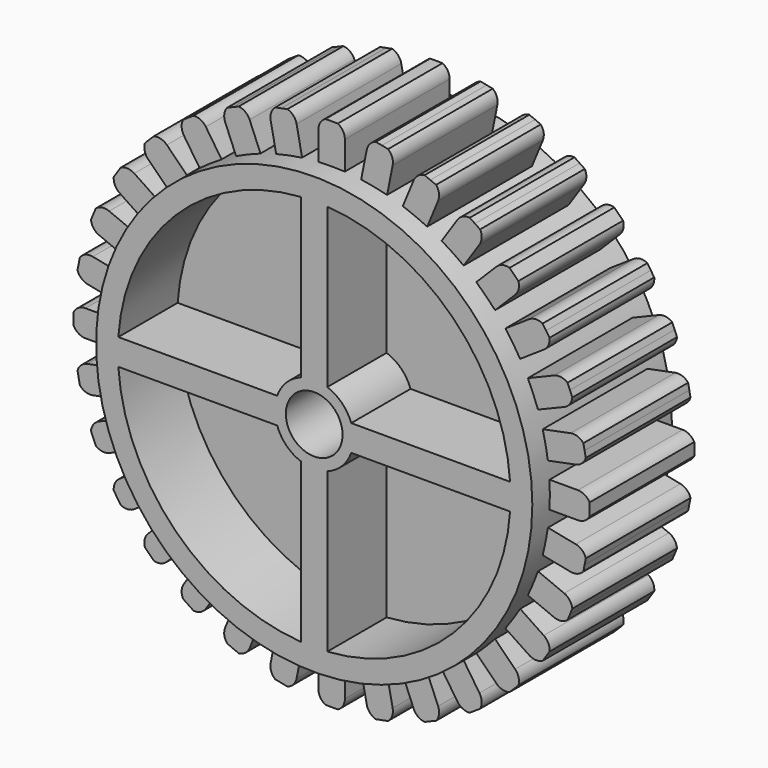
from build123d import *

# Parameters (mm, degrees)
F0_R      = 50
F1_DEPTH  = 20
F3_DEPTH  = 17
F5_DEPTH  = 17
F7_DEPTH  = 15
F8_R      = 9
F8_R_2    = 6.5
F9_DEPTH  = 20
F10_R     = 6.5
F11_DEPTH = 21


# Not quite as in the source:
# - a feature names something its author has since deleted; it is built from what else it names


with BuildPart() as f1:
    # F0 (on Front) → F1 (new body, symmetric)
    with BuildSketch(Plane.XZ):
        Circle(F0_R)
    extrude(amount=F1_DEPTH, both=True)

    # F2 (on face) → F3 (cut)
    with BuildSketch(Plane.XZ.offset(20)):
        with BuildLine():
            Line((-3, -3), (-44.8998886413, -3))
            ThreePointArc((-44.8998886413, -3), (-31.8198051534, -31.8198051534), (-3, -44.8998886413))
            Line((-3, -44.8998886413), (-3, -3))
        make_face()
        with BuildLine():
            ThreePointArc((-3, 44.8998886413), (-31.8198051534, 31.8198051534), (-44.8998886413, 3))
            Line((-44.8998886413, 3), (-3.2378670737, 3))
            Line((-3.2378670737, 3), (-3, 3.2378670737))
            Line((-3, 3.2378670737), (-3, 44.8998886413))
        make_face()
        Polygon((-3, 3.2378670737), (-3.2378670737, 3), (-3, 3), align=None)
        with BuildLine():
            ThreePointArc((44.8998886413, 3), (31.8198051534, 31.8198051534), (3, 44.8998886413))
            Line((3, 44.8998886413), (3, 3))
            Line((3, 3), (44.8998886413, 3))
        make_face()
        with BuildLine():
            Line((44.8998886413, -3), (3, -3))
            Line((3, -3), (3, -44.8998886413))
            ThreePointArc((3, -44.8998886413), (31.8198051534, -31.8198051534), (44.8998886413, -3))
        make_face()
    extrude(amount=-F3_DEPTH, mode=Mode.SUBTRACT)

    # F4 (on face) → F5 (cut)
    with BuildSketch(Plane(origin=(0, 20, 0), x_dir=(-1, 0, 0), z_dir=(0, 1, 0))):
        with BuildLine():
            Line((3, -3), (3, -44.8998886413))
            ThreePointArc((3, -44.8998886413), (31.8198051534, -31.8198051534), (44.8998886413, -3))
            Line((44.8998886413, -3), (3, -3))
        make_face()
        with BuildLine():
            Line((3, 3), (44.8998886413, 3))
            ThreePointArc((44.8998886413, 3), (31.8198051534, 31.8198051534), (3, 44.8998886413))
            Line((3, 44.8998886413), (3, 3))
        make_face()
        with BuildLine():
            ThreePointArc((-44.8998886413, -3), (-31.8198051534, -31.8198051534), (-3, -44.8998886413))
            Line((-3, -44.8998886413), (-3, -3))
            Line((-3, -3), (-44.8998886413, -3))
        make_face()
        with BuildLine():
            Line((-44.8998886413, 3), (-3, 3))
            Line((-3, 3), (-3, 44.8998886413))
            ThreePointArc((-3, 44.8998886413), (-31.8198051534, 31.8198051534), (-44.8998886413, 3))
        make_face()
    extrude(amount=-F5_DEPTH, mode=Mode.SUBTRACT)

    # F6 (on Front) → F7 (join, symmetric)
    with BuildSketch(Plane.XZ):
        with BuildLine():
            Line((-3.0323624939, 56.4412474632), (-3.0323624939, 49.947373569))
            Line((-3.0323624939, 49.947373569), (0, 49.947373569))
            Line((0, 49.947373569), (3.0323624939, 49.947373569))
            Line((3.0323624939, 49.947373569), (3.0323624939, 56.4412474632))
            ThreePointArc((3.0323624939, 56.4412474632), (2.5992583475, 58.0030023535), (1.4236640997, 59.1186347766))
            Line((1.4236640997, 59.1186347766), (0, 59.1186347766))
            Line((0, 59.1186347766), (-1.4236640997, 59.1186347766))
            ThreePointArc((-1.4236640997, 59.1186347766), (-2.5992583475, 58.0030023535), (-3.0323624939, 56.4412474632))
        make_face()
        with BuildLine():
            Line((-13.9852376415, 54.7651601441), (-12.7183456923, 48.3960642159))
            Line((-12.7183456923, 48.3960642159), (-9.7442491934, 48.9876487913))
            Line((-9.7442491934, 48.9876487913), (-6.7701526945, 49.5792333667))
            Line((-6.7701526945, 49.5792333667), (-8.0370446437, 55.9483292949))
            ThreePointArc((-8.0370446437, 55.9483292949), (-8.7665100798, 57.3955810756), (-10.1371647025, 58.2604298741))
            Line((-10.1371647025, 58.2604298741), (-11.5334734957, 57.9826867864))
            Line((-11.5334734957, 57.9826867864), (-12.9297822889, 57.7049436988))
            ThreePointArc((-12.9297822889, 57.7049436988), (-13.8651387343, 56.3814007795), (-13.9852376415, 54.7651601441))
        make_face()
        with BuildLine():
            Line((-24.4006679495, 50.9844784333), (-21.9155699983, 44.9849212558))
            Line((-21.9155699983, 44.9849212558), (-19.114032355, 46.1453561431))
            Line((-19.114032355, 46.1453561431), (-16.3124947117, 47.3057910305))
            Line((-16.3124947117, 47.3057910305), (-18.7975926629, 53.305348208))
            ThreePointArc((-18.7975926629, 53.305348208), (-19.7953864411, 54.5824798047), (-21.3084279502, 55.1633093243))
            Line((-21.3084279502, 55.1633093243), (-22.6237220731, 54.6184966601))
            Line((-22.6237220731, 54.6184966601), (-23.9390161959, 54.0736839959))
            ThreePointArc((-23.9390161959, 54.0736839959), (-24.5981896151, 52.5930935926), (-24.4006679495, 50.9844784333))
        make_face()
        with BuildLine():
            Line((-33.8783942723, 45.2444918088), (-30.2705912396, 39.8450329996))
            Line((-30.2705912396, 39.8450329996), (-27.7492739725, 41.529723337))
            Line((-27.7492739725, 41.529723337), (-25.2279567053, 43.2144136743))
            Line((-25.2279567053, 43.2144136743), (-28.8357597379, 48.6138724835))
            ThreePointArc((-28.8357597379, 48.6138724835), (-30.0635372029, 49.6718044451), (-31.6608202616, 49.9462937332))
            Line((-31.6608202616, 49.9462937332), (-32.8445536986, 49.1553483376))
            Line((-32.8445536986, 49.1553483376), (-34.0282871357, 48.364402942))
            ThreePointArc((-34.0282871357, 48.364402942), (-34.3859458639, 46.7836633135), (-33.8783942723, 45.2444918088))
        make_face()
        with BuildLine():
            Line((-42.0541929024, 37.7657847374), (-37.4623306356, 33.1739224706))
            Line((-37.4623306356, 33.1739224706), (-35.3181265531, 35.3181265531))
            Line((-35.3181265531, 35.3181265531), (-33.1739224706, 37.4623306356))
            Line((-33.1739224706, 37.4623306356), (-37.7657847374, 42.0541929024))
            ThreePointArc((-37.7657847374, 42.0541929024), (-39.1763630898, 42.852269497), (-40.796505006, 42.809870084))
            Line((-40.796505006, 42.809870084), (-41.803187545, 41.803187545))
            Line((-41.803187545, 41.803187545), (-42.809870084, 40.796505006))
            ThreePointArc((-42.809870084, 40.796505006), (-42.852269497, 39.1763630898), (-42.0541929024, 37.7657847374))
        make_face()
        with BuildLine():
            Line((-48.6138724835, 28.8357597379), (-43.2144136743, 25.2279567053))
            Line((-43.2144136743, 25.2279567053), (-41.529723337, 27.7492739725))
            Line((-41.529723337, 27.7492739725), (-39.8450329996, 30.2705912396))
            Line((-39.8450329996, 30.2705912396), (-45.2444918088, 33.8783942723))
            ThreePointArc((-45.2444918088, 33.8783942723), (-46.7836633135, 34.3859458639), (-48.364402942, 34.0282871357))
            Line((-48.364402942, 34.0282871357), (-49.1553483376, 32.8445536986))
            Line((-49.1553483376, 32.8445536986), (-49.9462937332, 31.6608202616))
            ThreePointArc((-49.9462937332, 31.6608202616), (-49.6718044451, 30.0635372029), (-48.6138724835, 28.8357597379))
        make_face()
        with BuildLine():
            Line((-53.305348208, 18.7975926629), (-47.3057910305, 16.3124947117))
            Line((-47.3057910305, 16.3124947117), (-46.1453561431, 19.114032355))
            Line((-46.1453561431, 19.114032355), (-44.9849212558, 21.9155699983))
            Line((-44.9849212558, 21.9155699983), (-50.9844784333, 24.4006679495))
            ThreePointArc((-50.9844784333, 24.4006679495), (-52.5930935926, 24.5981896151), (-54.0736839959, 23.9390161959))
            Line((-54.0736839959, 23.9390161959), (-54.6184966601, 22.6237220731))
            Line((-54.6184966601, 22.6237220731), (-55.1633093243, 21.3084279502))
            ThreePointArc((-55.1633093243, 21.3084279502), (-54.5824798047, 19.7953864411), (-53.305348208, 18.7975926629))
        make_face()
        with BuildLine():
            Line((-55.9483292949, 8.0370446437), (-49.5792333667, 6.7701526945))
            Line((-49.5792333667, 6.7701526945), (-48.9876487913, 9.7442491934))
            Line((-48.9876487913, 9.7442491934), (-48.3960642159, 12.7183456923))
            Line((-48.3960642159, 12.7183456923), (-54.7651601441, 13.9852376415))
            ThreePointArc((-54.7651601441, 13.9852376415), (-56.3814007795, 13.8651387343), (-57.7049436988, 12.9297822889))
            Line((-57.7049436988, 12.9297822889), (-57.9826867864, 11.5334734957))
            Line((-57.9826867864, 11.5334734957), (-58.2604298741, 10.1371647025))
            ThreePointArc((-58.2604298741, 10.1371647025), (-57.3955810756, 8.7665100798), (-55.9483292949, 8.0370446437))
        make_face()
        with BuildLine():
            Line((-56.4412474632, -3.0323624939), (-49.947373569, -3.0323624939))
            Line((-49.947373569, -3.0323624939), (-49.947373569, 0))
            Line((-49.947373569, 0), (-49.947373569, 3.0323624939))
            Line((-49.947373569, 3.0323624939), (-56.4412474632, 3.0323624939))
            ThreePointArc((-56.4412474632, 3.0323624939), (-58.0030023535, 2.5992583475), (-59.1186347766, 1.4236640997))
            Line((-59.1186347766, 1.4236640997), (-59.1186347766, 0))
            Line((-59.1186347766, 0), (-59.1186347766, -1.4236640997))
            ThreePointArc((-59.1186347766, -1.4236640997), (-58.0030023535, -2.5992583475), (-56.4412474632, -3.0323624939))
        make_face()
        with BuildLine():
            Line((-54.7651601441, -13.9852376415), (-48.3960642159, -12.7183456923))
            Line((-48.3960642159, -12.7183456923), (-48.9876487913, -9.7442491934))
            Line((-48.9876487913, -9.7442491934), (-49.5792333667, -6.7701526945))
            Line((-49.5792333667, -6.7701526945), (-55.9483292949, -8.0370446437))
            ThreePointArc((-55.9483292949, -8.0370446437), (-57.3955810756, -8.7665100798), (-58.2604298741, -10.1371647025))
            Line((-58.2604298741, -10.1371647025), (-57.9826867864, -11.5334734957))
            Line((-57.9826867864, -11.5334734957), (-57.7049436988, -12.9297822889))
            ThreePointArc((-57.7049436988, -12.9297822889), (-56.3814007795, -13.8651387343), (-54.7651601441, -13.9852376415))
        make_face()
        with BuildLine():
            Line((-50.9844784333, -24.4006679495), (-44.9849212558, -21.9155699983))
            Line((-44.9849212558, -21.9155699983), (-46.1453561431, -19.114032355))
            Line((-46.1453561431, -19.114032355), (-47.3057910305, -16.3124947117))
            Line((-47.3057910305, -16.3124947117), (-53.305348208, -18.7975926629))
            ThreePointArc((-53.305348208, -18.7975926629), (-54.5824798047, -19.7953864411), (-55.1633093243, -21.3084279502))
            Line((-55.1633093243, -21.3084279502), (-54.6184966601, -22.6237220731))
            Line((-54.6184966601, -22.6237220731), (-54.0736839959, -23.9390161959))
            ThreePointArc((-54.0736839959, -23.9390161959), (-52.5930935926, -24.5981896151), (-50.9844784333, -24.4006679495))
        make_face()
        with BuildLine():
            Line((-45.2444918088, -33.8783942723), (-39.8450329996, -30.2705912396))
            Line((-39.8450329996, -30.2705912396), (-41.529723337, -27.7492739725))
            Line((-41.529723337, -27.7492739725), (-43.2144136743, -25.2279567053))
            Line((-43.2144136743, -25.2279567053), (-48.6138724835, -28.8357597379))
            ThreePointArc((-48.6138724835, -28.8357597379), (-49.6718044451, -30.0635372029), (-49.9462937332, -31.6608202616))
            Line((-49.9462937332, -31.6608202616), (-49.1553483376, -32.8445536986))
            Line((-49.1553483376, -32.8445536986), (-48.364402942, -34.0282871357))
            ThreePointArc((-48.364402942, -34.0282871357), (-46.7836633135, -34.3859458639), (-45.2444918088, -33.8783942723))
        make_face()
        with BuildLine():
            Line((-37.7657847374, -42.0541929024), (-33.1739224706, -37.4623306356))
            Line((-33.1739224706, -37.4623306356), (-35.3181265531, -35.3181265531))
            Line((-35.3181265531, -35.3181265531), (-37.4623306356, -33.1739224706))
            Line((-37.4623306356, -33.1739224706), (-42.0541929024, -37.7657847374))
            ThreePointArc((-42.0541929024, -37.7657847374), (-42.852269497, -39.1763630898), (-42.809870084, -40.796505006))
            Line((-42.809870084, -40.796505006), (-41.803187545, -41.803187545))
            Line((-41.803187545, -41.803187545), (-40.796505006, -42.809870084))
            ThreePointArc((-40.796505006, -42.809870084), (-39.1763630898, -42.852269497), (-37.7657847374, -42.0541929024))
        make_face()
        with BuildLine():
            Line((-28.8357597379, -48.6138724835), (-25.2279567053, -43.2144136743))
            Line((-25.2279567053, -43.2144136743), (-27.7492739725, -41.529723337))
            Line((-27.7492739725, -41.529723337), (-30.2705912396, -39.8450329996))
            Line((-30.2705912396, -39.8450329996), (-33.8783942723, -45.2444918088))
            ThreePointArc((-33.8783942723, -45.2444918088), (-34.3859458639, -46.7836633135), (-34.0282871357, -48.364402942))
            Line((-34.0282871357, -48.364402942), (-32.8445536986, -49.1553483376))
            Line((-32.8445536986, -49.1553483376), (-31.6608202616, -49.9462937332))
            ThreePointArc((-31.6608202616, -49.9462937332), (-30.0635372029, -49.6718044451), (-28.8357597379, -48.6138724835))
        make_face()
        with BuildLine():
            Line((-18.7975926629, -53.305348208), (-16.3124947117, -47.3057910305))
            Line((-16.3124947117, -47.3057910305), (-19.114032355, -46.1453561431))
            Line((-19.114032355, -46.1453561431), (-21.9155699983, -44.9849212558))
            Line((-21.9155699983, -44.9849212558), (-24.4006679495, -50.9844784333))
            ThreePointArc((-24.4006679495, -50.9844784333), (-24.5981896151, -52.5930935926), (-23.9390161959, -54.0736839959))
            Line((-23.9390161959, -54.0736839959), (-22.6237220731, -54.6184966601))
            Line((-22.6237220731, -54.6184966601), (-21.3084279502, -55.1633093243))
            ThreePointArc((-21.3084279502, -55.1633093243), (-19.7953864411, -54.5824798047), (-18.7975926629, -53.305348208))
        make_face()
        with BuildLine():
            Line((-8.0370446437, -55.9483292949), (-6.7701526945, -49.5792333667))
            Line((-6.7701526945, -49.5792333667), (-9.7442491934, -48.9876487913))
            Line((-9.7442491934, -48.9876487913), (-12.7183456923, -48.3960642159))
            Line((-12.7183456923, -48.3960642159), (-13.9852376415, -54.7651601441))
            ThreePointArc((-13.9852376415, -54.7651601441), (-13.8651387343, -56.3814007795), (-12.9297822889, -57.7049436988))
            Line((-12.9297822889, -57.7049436988), (-11.5334734957, -57.9826867864))
            Line((-11.5334734957, -57.9826867864), (-10.1371647025, -58.2604298741))
            ThreePointArc((-10.1371647025, -58.2604298741), (-8.7665100798, -57.3955810756), (-8.0370446437, -55.9483292949))
        make_face()
        with BuildLine():
            Line((3.0323624939, -56.4412474632), (3.0323624939, -49.947373569))
            Line((3.0323624939, -49.947373569), (0, -49.947373569))
            Line((0, -49.947373569), (-3.0323624939, -49.947373569))
            Line((-3.0323624939, -49.947373569), (-3.0323624939, -56.4412474632))
            ThreePointArc((-3.0323624939, -56.4412474632), (-2.5992583475, -58.0030023535), (-1.4236640997, -59.1186347766))
            Line((-1.4236640997, -59.1186347766), (0, -59.1186347766))
            Line((0, -59.1186347766), (1.4236640997, -59.1186347766))
            ThreePointArc((1.4236640997, -59.1186347766), (2.5992583475, -58.0030023535), (3.0323624939, -56.4412474632))
        make_face()
        with BuildLine():
            Line((13.9852376415, -54.7651601441), (12.7183456923, -48.3960642159))
            Line((12.7183456923, -48.3960642159), (9.7442491934, -48.9876487913))
            Line((9.7442491934, -48.9876487913), (6.7701526945, -49.5792333667))
            Line((6.7701526945, -49.5792333667), (8.0370446437, -55.9483292949))
            ThreePointArc((8.0370446437, -55.9483292949), (8.7665100798, -57.3955810756), (10.1371647025, -58.2604298741))
            Line((10.1371647025, -58.2604298741), (11.5334734957, -57.9826867864))
            Line((11.5334734957, -57.9826867864), (12.9297822889, -57.7049436988))
            ThreePointArc((12.9297822889, -57.7049436988), (13.8651387343, -56.3814007795), (13.9852376415, -54.7651601441))
        make_face()
        with BuildLine():
            Line((24.4006679495, -50.9844784333), (21.9155699983, -44.9849212558))
            Line((21.9155699983, -44.9849212558), (19.114032355, -46.1453561431))
            Line((19.114032355, -46.1453561431), (16.3124947117, -47.3057910305))
            Line((16.3124947117, -47.3057910305), (18.7975926629, -53.305348208))
            ThreePointArc((18.7975926629, -53.305348208), (19.7953864411, -54.5824798047), (21.3084279502, -55.1633093243))
            Line((21.3084279502, -55.1633093243), (22.6237220731, -54.6184966601))
            Line((22.6237220731, -54.6184966601), (23.9390161959, -54.0736839959))
            ThreePointArc((23.9390161959, -54.0736839959), (24.5981896151, -52.5930935926), (24.4006679495, -50.9844784333))
        make_face()
        with BuildLine():
            Line((33.8783942723, -45.2444918088), (30.2705912396, -39.8450329996))
            Line((30.2705912396, -39.8450329996), (27.7492739725, -41.529723337))
            Line((27.7492739725, -41.529723337), (25.2279567053, -43.2144136743))
            Line((25.2279567053, -43.2144136743), (28.8357597379, -48.6138724835))
            ThreePointArc((28.8357597379, -48.6138724835), (30.0635372029, -49.6718044451), (31.6608202616, -49.9462937332))
            Line((31.6608202616, -49.9462937332), (32.8445536986, -49.1553483376))
            Line((32.8445536986, -49.1553483376), (34.0282871357, -48.364402942))
            ThreePointArc((34.0282871357, -48.364402942), (34.3859458639, -46.7836633135), (33.8783942723, -45.2444918088))
        make_face()
        with BuildLine():
            Line((42.0541929024, -37.7657847374), (37.4623306356, -33.1739224706))
            Line((37.4623306356, -33.1739224706), (35.3181265531, -35.3181265531))
            Line((35.3181265531, -35.3181265531), (33.1739224706, -37.4623306356))
            Line((33.1739224706, -37.4623306356), (37.7657847374, -42.0541929024))
            ThreePointArc((37.7657847374, -42.0541929024), (39.1763630898, -42.852269497), (40.796505006, -42.809870084))
            Line((40.796505006, -42.809870084), (41.803187545, -41.803187545))
            Line((41.803187545, -41.803187545), (42.809870084, -40.796505006))
            ThreePointArc((42.809870084, -40.796505006), (42.852269497, -39.1763630898), (42.0541929024, -37.7657847374))
        make_face()
        with BuildLine():
            Line((48.6138724835, -28.8357597379), (43.2144136743, -25.2279567053))
            Line((43.2144136743, -25.2279567053), (41.529723337, -27.7492739725))
            Line((41.529723337, -27.7492739725), (39.8450329996, -30.2705912396))
            Line((39.8450329996, -30.2705912396), (45.2444918088, -33.8783942723))
            ThreePointArc((45.2444918088, -33.8783942723), (46.7836633135, -34.3859458639), (48.364402942, -34.0282871357))
            Line((48.364402942, -34.0282871357), (49.1553483376, -32.8445536986))
            Line((49.1553483376, -32.8445536986), (49.9462937332, -31.6608202616))
            ThreePointArc((49.9462937332, -31.6608202616), (49.6718044451, -30.0635372029), (48.6138724835, -28.8357597379))
        make_face()
        with BuildLine():
            Line((53.305348208, -18.7975926629), (47.3057910305, -16.3124947117))
            Line((47.3057910305, -16.3124947117), (46.1453561431, -19.114032355))
            Line((46.1453561431, -19.114032355), (44.9849212558, -21.9155699983))
            Line((44.9849212558, -21.9155699983), (50.9844784333, -24.4006679495))
            ThreePointArc((50.9844784333, -24.4006679495), (52.5930935926, -24.5981896151), (54.0736839959, -23.9390161959))
            Line((54.0736839959, -23.9390161959), (54.6184966601, -22.6237220731))
            Line((54.6184966601, -22.6237220731), (55.1633093243, -21.3084279502))
            ThreePointArc((55.1633093243, -21.3084279502), (54.5824798047, -19.7953864411), (53.305348208, -18.7975926629))
        make_face()
        with BuildLine():
            Line((55.9483292949, -8.0370446437), (49.5792333667, -6.7701526945))
            Line((49.5792333667, -6.7701526945), (48.9876487913, -9.7442491934))
            Line((48.9876487913, -9.7442491934), (48.3960642159, -12.7183456923))
            Line((48.3960642159, -12.7183456923), (54.7651601441, -13.9852376415))
            ThreePointArc((54.7651601441, -13.9852376415), (56.3814007795, -13.8651387343), (57.7049436988, -12.9297822889))
            Line((57.7049436988, -12.9297822889), (57.9826867864, -11.5334734957))
            Line((57.9826867864, -11.5334734957), (58.2604298741, -10.1371647025))
            ThreePointArc((58.2604298741, -10.1371647025), (57.3955810756, -8.7665100798), (55.9483292949, -8.0370446437))
        make_face()
        with BuildLine():
            Line((56.4412474632, 3.0323624939), (49.947373569, 3.0323624939))
            Line((49.947373569, 3.0323624939), (49.947373569, 0))
            Line((49.947373569, 0), (49.947373569, -3.0323624939))
            Line((49.947373569, -3.0323624939), (56.4412474632, -3.0323624939))
            ThreePointArc((56.4412474632, -3.0323624939), (58.0030023535, -2.5992583475), (59.1186347766, -1.4236640997))
            Line((59.1186347766, -1.4236640997), (59.1186347766, 0))
            Line((59.1186347766, 0), (59.1186347766, 1.4236640997))
            ThreePointArc((59.1186347766, 1.4236640997), (58.0030023535, 2.5992583475), (56.4412474632, 3.0323624939))
        make_face()
        with BuildLine():
            Line((54.7651601441, 13.9852376415), (48.3960642159, 12.7183456923))
            Line((48.3960642159, 12.7183456923), (48.9876487913, 9.7442491934))
            Line((48.9876487913, 9.7442491934), (49.5792333667, 6.7701526945))
            Line((49.5792333667, 6.7701526945), (55.9483292949, 8.0370446437))
            ThreePointArc((55.9483292949, 8.0370446437), (57.3955810756, 8.7665100798), (58.2604298741, 10.1371647025))
            Line((58.2604298741, 10.1371647025), (57.9826867864, 11.5334734957))
            Line((57.9826867864, 11.5334734957), (57.7049436988, 12.9297822889))
            ThreePointArc((57.7049436988, 12.9297822889), (56.3814007795, 13.8651387343), (54.7651601441, 13.9852376415))
        make_face()
        with BuildLine():
            Line((50.9844784333, 24.4006679495), (44.9849212558, 21.9155699983))
            Line((44.9849212558, 21.9155699983), (46.1453561431, 19.114032355))
            Line((46.1453561431, 19.114032355), (47.3057910305, 16.3124947117))
            Line((47.3057910305, 16.3124947117), (53.305348208, 18.7975926629))
            ThreePointArc((53.305348208, 18.7975926629), (54.5824798047, 19.7953864411), (55.1633093243, 21.3084279502))
            Line((55.1633093243, 21.3084279502), (54.6184966601, 22.6237220731))
            Line((54.6184966601, 22.6237220731), (54.0736839959, 23.9390161959))
            ThreePointArc((54.0736839959, 23.9390161959), (52.5930935926, 24.5981896151), (50.9844784333, 24.4006679495))
        make_face()
        with BuildLine():
            Line((45.2444918088, 33.8783942723), (39.8450329996, 30.2705912396))
            Line((39.8450329996, 30.2705912396), (41.529723337, 27.7492739725))
            Line((41.529723337, 27.7492739725), (43.2144136743, 25.2279567053))
            Line((43.2144136743, 25.2279567053), (48.6138724835, 28.8357597379))
            ThreePointArc((48.6138724835, 28.8357597379), (49.6718044451, 30.0635372029), (49.9462937332, 31.6608202616))
            Line((49.9462937332, 31.6608202616), (49.1553483376, 32.8445536986))
            Line((49.1553483376, 32.8445536986), (48.364402942, 34.0282871357))
            ThreePointArc((48.364402942, 34.0282871357), (46.7836633135, 34.3859458639), (45.2444918088, 33.8783942723))
        make_face()
        with BuildLine():
            Line((37.7657847374, 42.0541929024), (33.1739224706, 37.4623306356))
            Line((33.1739224706, 37.4623306356), (35.3181265531, 35.3181265531))
            Line((35.3181265531, 35.3181265531), (37.4623306356, 33.1739224706))
            Line((37.4623306356, 33.1739224706), (42.0541929024, 37.7657847374))
            ThreePointArc((42.0541929024, 37.7657847374), (42.852269497, 39.1763630898), (42.809870084, 40.796505006))
            Line((42.809870084, 40.796505006), (41.803187545, 41.803187545))
            Line((41.803187545, 41.803187545), (40.796505006, 42.809870084))
            ThreePointArc((40.796505006, 42.809870084), (39.1763630898, 42.852269497), (37.7657847374, 42.0541929024))
        make_face()
        with BuildLine():
            Line((28.8357597379, 48.6138724835), (25.2279567053, 43.2144136743))
            Line((25.2279567053, 43.2144136743), (27.7492739725, 41.529723337))
            Line((27.7492739725, 41.529723337), (30.2705912396, 39.8450329996))
            Line((30.2705912396, 39.8450329996), (33.8783942723, 45.2444918088))
            ThreePointArc((33.8783942723, 45.2444918088), (34.3859458639, 46.7836633135), (34.0282871357, 48.364402942))
            Line((34.0282871357, 48.364402942), (32.8445536986, 49.1553483376))
            Line((32.8445536986, 49.1553483376), (31.6608202616, 49.9462937332))
            ThreePointArc((31.6608202616, 49.9462937332), (30.0635372029, 49.6718044451), (28.8357597379, 48.6138724835))
        make_face()
        with BuildLine():
            Line((18.7975926629, 53.305348208), (16.3124947117, 47.3057910305))
            Line((16.3124947117, 47.3057910305), (19.114032355, 46.1453561431))
            Line((19.114032355, 46.1453561431), (21.9155699983, 44.9849212558))
            Line((21.9155699983, 44.9849212558), (24.4006679495, 50.9844784333))
            ThreePointArc((24.4006679495, 50.9844784333), (24.5981896151, 52.5930935926), (23.9390161959, 54.0736839959))
            Line((23.9390161959, 54.0736839959), (22.6237220731, 54.6184966601))
            Line((22.6237220731, 54.6184966601), (21.3084279502, 55.1633093243))
            ThreePointArc((21.3084279502, 55.1633093243), (19.7953864411, 54.5824798047), (18.7975926629, 53.305348208))
        make_face()
        with BuildLine():
            Line((8.0370446437, 55.9483292949), (6.7701526945, 49.5792333667))
            Line((6.7701526945, 49.5792333667), (9.7442491934, 48.9876487913))
            Line((9.7442491934, 48.9876487913), (12.7183456923, 48.3960642159))
            Line((12.7183456923, 48.3960642159), (13.9852376415, 54.7651601441))
            ThreePointArc((13.9852376415, 54.7651601441), (13.8651387343, 56.3814007795), (12.9297822889, 57.7049436988))
            Line((12.9297822889, 57.7049436988), (11.5334734957, 57.9826867864))
            Line((11.5334734957, 57.9826867864), (10.1371647025, 58.2604298741))
            ThreePointArc((10.1371647025, 58.2604298741), (8.7665100798, 57.3955810756), (8.0370446437, 55.9483292949))
        make_face()
    extrude(amount=F7_DEPTH, both=True)

    # F8 (on Front) → F9 (join, symmetric)
    with BuildSketch(Plane.XZ):
        Circle(F8_R)
        Circle(F8_R_2, mode=Mode.SUBTRACT)
    extrude(amount=F9_DEPTH, both=True)

    # F10 (on Front) → F11 (cut, symmetric)
    with BuildSketch(Plane.XZ):
        Circle(F10_R)
    extrude(amount=F11_DEPTH, both=True, mode=Mode.SUBTRACT)


solid = f1.part
